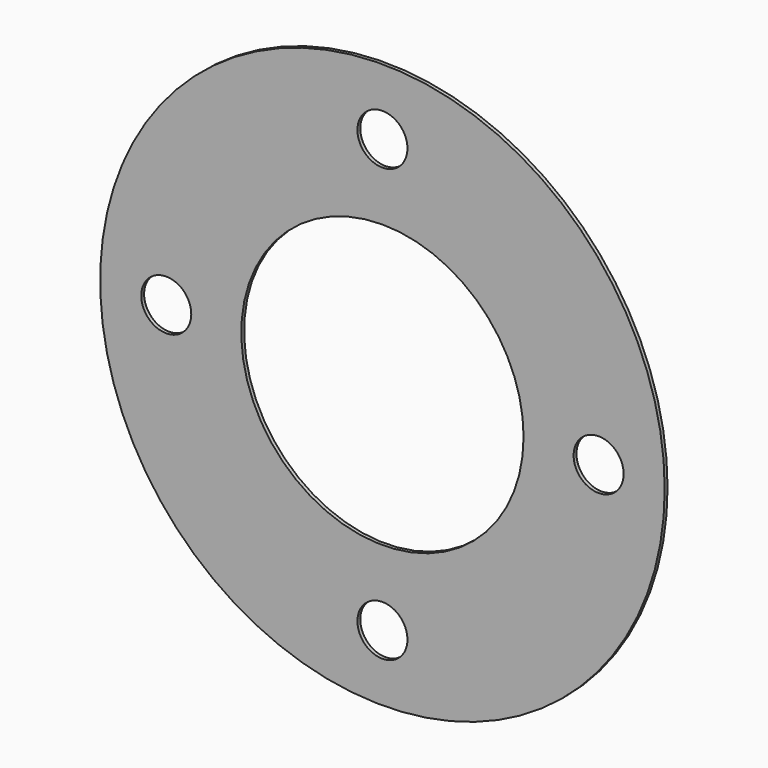
from build123d import *

# Parameters (mm, degrees)
F0_R     = 79
F1_DEPTH = 1


with BuildPart() as f1:
    # F0 (on Front) → F1 (new body)
    with BuildSketch(Plane.XZ):
        Circle(F0_R)
        with BuildLine():
            ThreePointArc((6.9882765021, 60.0950413223), (42.7799602618, 42.7799602618), (60.0950413223, 6.9882765021))
            ThreePointArc((60.0950413223, 6.9882765021), (65.3044400952, 5.0909090909), (67.5, 0))
            ThreePointArc((67.5, 0), (65.3044400952, -5.0909090909), (60.0950413223, -6.9882765021))
            ThreePointArc((60.0950413223, -6.9882765021), (42.7799602618, -42.7799602618), (6.9882765021, -60.0950413223))
            ThreePointArc((6.9882765021, -60.0950413223), (6.9970685117, -60.2974358305), (7, -60.5))
            ThreePointArc((7, -60.5), (-0.2025641695, -67.4970685117), (-6.9882765021, -60.0950413223))
            ThreePointArc((-6.9882765021, -60.0950413223), (-42.7799602618, -42.7799602618), (-60.0950413223, -6.9882765021))
            ThreePointArc((-60.0950413223, -6.9882765021), (-67.5, 0), (-60.0950413223, 6.9882765021))
            ThreePointArc((-60.0950413223, 6.9882765021), (-42.7799602618, 42.7799602618), (-6.9882765021, 60.0950413223))
            ThreePointArc((-6.9882765021, 60.0950413223), (-0.2025641695, 67.4970685117), (7, 60.5))
            ThreePointArc((7, 60.5), (6.9970685117, 60.2974358305), (6.9882765021, 60.0950413223))
        make_face(mode=Mode.SUBTRACT)
        with BuildLine():
            ThreePointArc((60.0950413223, -6.9882765021), (53.5, 0), (60.0950413223, 6.9882765021))
            ThreePointArc((60.0950413223, 6.9882765021), (42.7799602618, 42.7799602618), (6.9882765021, 60.0950413223))
            ThreePointArc((6.9882765021, 60.0950413223), (4.8044400952, 55.4090909091), (0, 53.5))
            ThreePointArc((0, 53.5), (-4.8044400952, 55.4090909091), (-6.9882765021, 60.0950413223))
            ThreePointArc((-6.9882765021, 60.0950413223), (-42.7799602618, 42.7799602618), (-60.0950413223, 6.9882765021))
            ThreePointArc((-60.0950413223, 6.9882765021), (-55.4090909091, 4.8044400952), (-53.5, 0))
            ThreePointArc((-53.5, 0), (-55.4090909091, -4.8044400952), (-60.0950413223, -6.9882765021))
            ThreePointArc((-60.0950413223, -6.9882765021), (-42.7799602618, -42.7799602618), (-6.9882765021, -60.0950413223))
            ThreePointArc((-6.9882765021, -60.0950413223), (0, -53.5), (6.9882765021, -60.0950413223))
            ThreePointArc((6.9882765021, -60.0950413223), (42.7799602618, -42.7799602618), (60.0950413223, -6.9882765021))
        make_face()
        with BuildLine():
            ThreePointArc((39.5, 0), (-27.9307178569, -27.9307178569), (0, 39.5))
            ThreePointArc((0, 39.5), (27.9307178569, 27.9307178569), (39.5, 0))
        make_face(mode=Mode.SUBTRACT)
    extrude(amount=F1_DEPTH)


solid = f1.part
